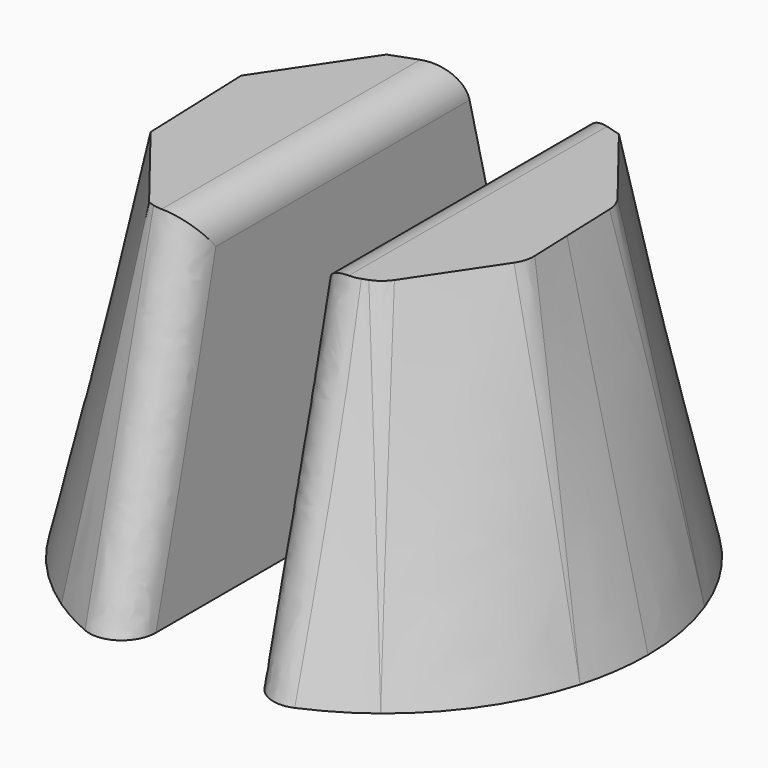
from build123d import *

# Parameters (mm, degrees)
F0_R     = 40
F5_W     = 17.9323302582
F5_H     = 58.3646646701
F6_DEPTH = 92.8
F7_R     = 5


with BuildPart() as f3:
    # F2 (on offset) → F3 section 0
    with BuildSketch(Plane.XY.offset(51.9)):
        Polygon((17.9732700356, -22.9228152642), (28.0143736566, -7.9805240452), (27.3549387144, 10.010056111), (16.2468469433, 24.1771350621), (-1.06698815, 29.1093701701), (-17.9732700356, 22.9228152642), (-28.0143736566, 7.9805240452), (-27.3549387144, -10.010056111), (-16.2468469433, -24.1771350621), (1.06698815, -29.1093701701), align=None)
    # F0 (on Top) → F3 section 1
    with BuildSketch(Plane.XY):
        Circle(F0_R)
    loft()

    # F5 (on offset) → F6 (cut)
    with BuildSketch(Plane.XZ.offset(-41.5)):
        with Locations((-0.0380412675, 24.9530088622)):
            Rectangle(F5_W, F5_H)
    extrude(amount=F6_DEPTH, mode=Mode.SUBTRACT)

    # F7
    f7_edges = [f3.edges().sort_by_distance(p)[0] for p in [
        (8.928124, 0.014656, 51.9),
        (-9.004206, -32.63119, 25.95596),
        (8.928124, -32.700734, 25.971852),
        (-9.004206, -0.017739, 51.9),
        (32.45945, 11.877962, 25.95),
        (33.241937, -9.469713, 25.95),
        (21.327134, -27.200279, 25.95),
    ]]
    fillet(f7_edges, radius=F7_R)


solid = f3.part
